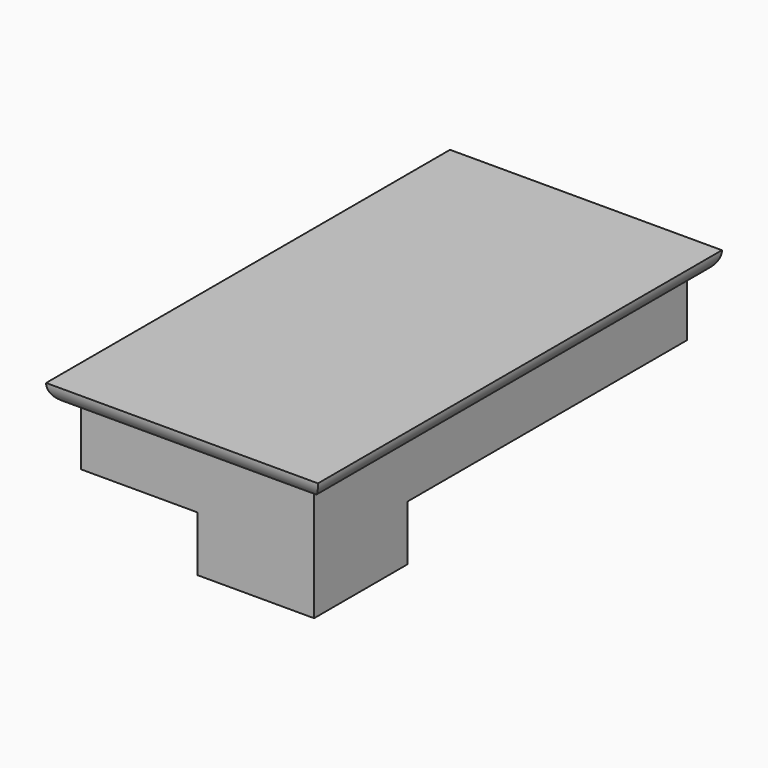
from build123d import *

# Parameters (mm, degrees)
F0_W     = 88.9
F0_H     = 165.1
F1_DEPTH = 6.35
F2_DEPTH = 25.4
F3_DEPTH = 50.8
F4_R     = 6.34999
F5_SIZE2 = 7.3323484187
F5_SIZE  = 12.7
F6_SIZE2 = 7.3323484187
F6_SIZE  = 12.7


# Not quite as in the source:
# - a fillet or chamfer is up to 0.001 mm smaller than in the source, because OpenCascade refuses the exact size


with BuildPart() as f1:
    # F0 (on Top) → F1 (new body)
    with BuildSketch(Plane.XY):
        with Locations((-44.4500000971, -25.0825021148)):
            Rectangle(F0_W, F0_H)
        Polygon((-82.5500000971, 13.0174978852), (-82.5500000971, 51.1174978852), (-44.4500000971, 51.1174978852), (-6.3500000971, 51.1174978852), (-6.3500000971, -63.1825021148), (-6.3500000971, -101.2825021148), (-44.4500000971, -101.2825021148), (-82.5500000971, -101.2825021148), align=None, mode=Mode.SUBTRACT)
        with BuildLine():
            Line((-6.3500000971, 51.1174978852), (-44.4500000971, 51.1174978852))
            Line((-44.4500000971, 51.1174978852), (-44.4500000971, 25.7174978852))
            ThreePointArc((-44.4500000971, 25.7174978852), (-48.169743976, 16.7372417642), (-57.1500000971, 13.0174978852))
            Line((-57.1500000971, 13.0174978852), (-82.5500000971, 13.0174978852))
            Line((-82.5500000971, 13.0174978852), (-82.5500000971, -101.2825021148))
            Line((-82.5500000971, -101.2825021148), (-44.4500000971, -101.2825021148))
            Line((-44.4500000971, -101.2825021148), (-44.4500000971, -75.8825021148))
            ThreePointArc((-44.4500000971, -75.8825021148), (-40.7302562182, -66.9022459937), (-31.7500000971, -63.1825021148))
            Line((-31.7500000971, -63.1825021148), (-6.3500000971, -63.1825021148))
            Line((-6.3500000971, -63.1825021148), (-6.3500000971, 51.1174978852))
        make_face()
        with BuildLine():
            Line((-6.3500000971, -101.2825021148), (-6.3500000971, -63.1825021148))
            Line((-6.3500000971, -63.1825021148), (-31.7500000971, -63.1825021148))
            ThreePointArc((-31.7500000971, -63.1825021148), (-40.7302562182, -66.9022459937), (-44.4500000971, -75.8825021148))
            Line((-44.4500000971, -75.8825021148), (-44.4500000971, -101.2825021148))
            Line((-44.4500000971, -101.2825021148), (-6.3500000971, -101.2825021148))
        make_face()
        with BuildLine():
            Line((-44.4500000971, 51.1174978852), (-82.5500000971, 51.1174978852))
            Line((-82.5500000971, 51.1174978852), (-82.5500000971, 13.0174978852))
            Line((-82.5500000971, 13.0174978852), (-57.1500000971, 13.0174978852))
            ThreePointArc((-57.1500000971, 13.0174978852), (-48.169743976, 16.7372417642), (-44.4500000971, 25.7174978852))
            Line((-44.4500000971, 25.7174978852), (-44.4500000971, 51.1174978852))
        make_face()
    extrude(amount=-F1_DEPTH)

    # F0 (on Top) → F2 (join)
    with BuildSketch(Plane.XY):
        with BuildLine():
            Line((-6.3500000971, 51.1174978852), (-44.4500000971, 51.1174978852))
            Line((-44.4500000971, 51.1174978852), (-44.4500000971, 25.7174978852))
            ThreePointArc((-44.4500000971, 25.7174978852), (-48.169743976, 16.7372417642), (-57.1500000971, 13.0174978852))
            Line((-57.1500000971, 13.0174978852), (-82.5500000971, 13.0174978852))
            Line((-82.5500000971, 13.0174978852), (-82.5500000971, -101.2825021148))
            Line((-82.5500000971, -101.2825021148), (-44.4500000971, -101.2825021148))
            Line((-44.4500000971, -101.2825021148), (-44.4500000971, -75.8825021148))
            ThreePointArc((-44.4500000971, -75.8825021148), (-40.7302562182, -66.9022459937), (-31.7500000971, -63.1825021148))
            Line((-31.7500000971, -63.1825021148), (-6.3500000971, -63.1825021148))
            Line((-6.3500000971, -63.1825021148), (-6.3500000971, 51.1174978852))
        make_face()
    extrude(amount=-F2_DEPTH)

    # F0 (on Top) → F3 (join)
    with BuildSketch(Plane.XY):
        with BuildLine():
            Line((-6.3500000971, -101.2825021148), (-6.3500000971, -63.1825021148))
            Line((-6.3500000971, -63.1825021148), (-31.7500000971, -63.1825021148))
            ThreePointArc((-31.7500000971, -63.1825021148), (-40.7302562182, -66.9022459937), (-44.4500000971, -75.8825021148))
            Line((-44.4500000971, -75.8825021148), (-44.4500000971, -101.2825021148))
            Line((-44.4500000971, -101.2825021148), (-6.3500000971, -101.2825021148))
        make_face()
        with BuildLine():
            Line((-44.4500000971, 51.1174978852), (-82.5500000971, 51.1174978852))
            Line((-82.5500000971, 51.1174978852), (-82.5500000971, 13.0174978852))
            Line((-82.5500000971, 13.0174978852), (-57.1500000971, 13.0174978852))
            ThreePointArc((-57.1500000971, 13.0174978852), (-48.169743976, 16.7372417642), (-44.4500000971, 25.7174978852))
            Line((-44.4500000971, 25.7174978852), (-44.4500000971, 51.1174978852))
        make_face()
    extrude(amount=-F3_DEPTH)

    # F4 (radius 6.35 in the source; OpenCascade refuses exactly that, so slightly less here)
    f4_edges = [f1.edges().sort_by_distance(p)[0] for p in [
        (-44.45, 57.467498, -6.35),
        (0, -25.082502, -6.35),
        (-44.45, -107.632502, -6.35),
        (-88.9, -25.082502, -6.35),
    ]]
    fillet(f4_edges, radius=F4_R)

    # F5
    f5_edges = [f1.edges().sort_by_distance(p)[0] for p in [
        (-6.35, -82.232502, -50.8),
        (-25.4, -101.282502, -50.8),
    ]]
    f5_side = f1.faces().sort_by_distance((-25.003958, -82.628544, -50.8))[0]
    chamfer(f5_edges, length=F5_SIZE, length2=F5_SIZE2, reference=f5_side)

    # F6
    f6_edges = [f1.edges().sort_by_distance(p)[0] for p in [
        (-82.55, 32.067498, -50.8),
        (-63.5, 51.117498, -50.8),
    ]]
    chamfer(f6_edges, length=F6_SIZE, length2=F6_SIZE2)


solid = f1.part
